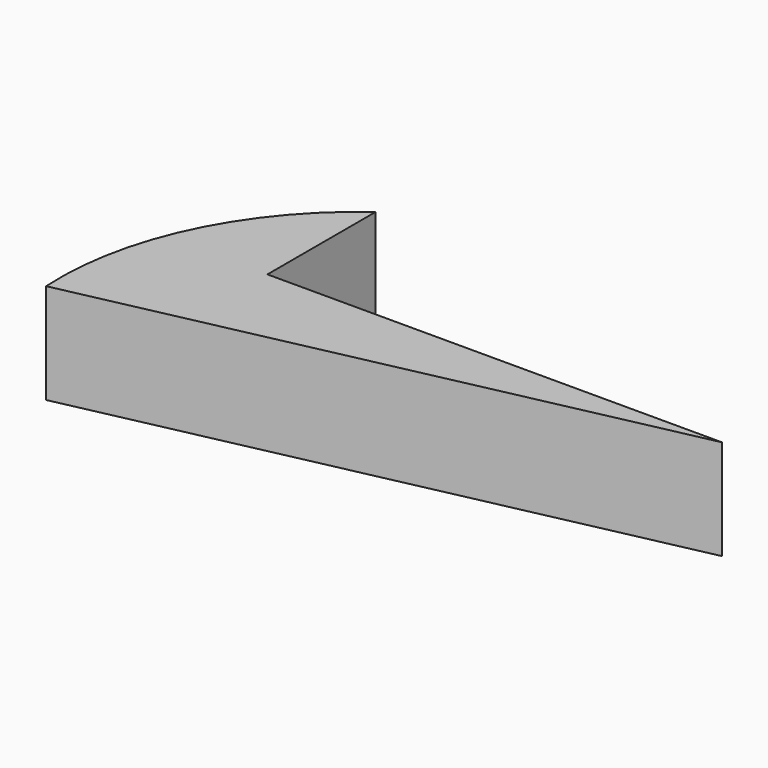
from build123d import *

# Parameters (mm, degrees)
F1_DEPTH = 25.4
F2_W     = 115.2222603559
F2_H     = 34.2616252165
F3_DEPTH = 25.4


# Not quite as in the source:
# - a feature of the source that left no trace in its solid (it failed there, or was rolled back) is left out


with BuildPart() as f1:
    # F0 (on Top) → F1 (new body)
    with BuildSketch(Plane.XY):
        with BuildLine():
            ThreePointArc((-115.2222603559, 34.4368517399), (-139.1213542265, 5.6159757036), (-146.2818682194, -31.1336722225))
            Line((-146.2818682194, -31.1336722225), (-115.2222603559, 34.4368517399))
        make_face()
        Polygon((-115.2222603559, 34.4368517399), (-146.2818682194, -31.1336722225), (0, 0.1752265234), align=None)
    extrude(amount=F1_DEPTH)

    # F2 (on face) → F3 (cut)
    with BuildSketch(Plane.XY.offset(25.4)):
        with Locations((-57.611130178, 17.3060391317)):
            Rectangle(F2_W, F2_H)
    extrude(amount=-F3_DEPTH, mode=Mode.SUBTRACT)


solid = f1.part
